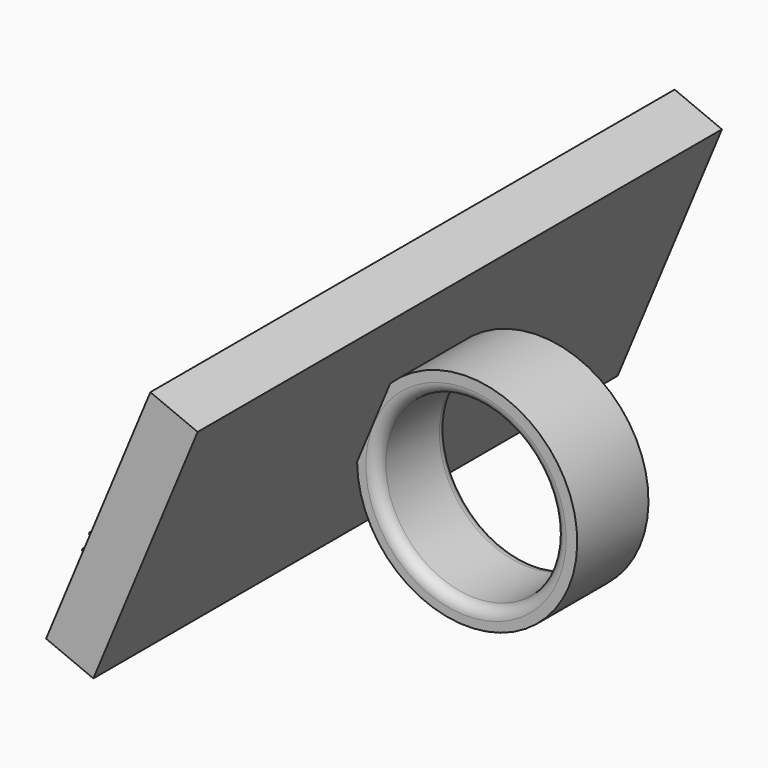
from build123d import *

# Parameters (mm, degrees)
F0_R           = 10.16
F1_DEPTH       = 10.16
F2_R           = 1.27
F3_R           = 1.27
F5_W           = 74.7877769172
F5_H           = 31.0049764812
F6_DEPTH       = 5.842
F7_TEXT_SIZE   = 4.4080810363
F7_TEXT_SIZE_2 = 4.4057197455
F7_TEXT_SIZE_3 = 4.3735069792
F7_TEXT_SIZE_4 = 4.335331121
F7_TEXT_SIZE_5 = 4.2736875912
F7_TEXT_SIZE_6 = 4.2982167037
F7_TEXT_SIZE_7 = 4.3517716727
F7_TEXT_SIZE_8 = 4.3960835481
F8_DEPTH       = 1.524


# Not quite as in the source:
# - Text() gives the source's letters only with a copy of the font that has no kerning and outlines rounded to 1/6400 em; it was checked with that copy


with BuildPart() as f1:
    # F0 (on Front) → F1 (new body)
    with BuildSketch(Plane.XZ):
        with BuildLine():
            Line((-8.6544063684, 9.0933511978), (-12.4330554948, 0))
            ThreePointArc((-12.4330554948, 0), (11.730902079, -4.7093204288), (-8.6544063684, 9.0933511978))
        make_face()
        Circle(F0_R, mode=Mode.SUBTRACT)
    extrude(amount=F1_DEPTH)

    # F2
    f2_edges = [f1.edges().sort_by_distance(p)[0] for p in [
        (-10.16, 0, 0),
    ]]
    fillet(f2_edges, radius=F2_R)

    # F3
    f3_edges = [f1.edges().sort_by_distance(p)[0] for p in [
        (-10.16, -10.16, 0),
    ]]
    fillet(f3_edges, radius=F3_R)

    # F5 (on offset) → F6 (join)
    with BuildSketch(Plane(origin=(-10.6023181655, 0, 4.4056849232), x_dir=(0, -1, 0), z_dir=(-0.9234459488, 0, 0.3837285234))):
        with Locations((5.2367541939, 0)):
            Rectangle(F5_W, F5_H)
    extrude(amount=F6_DEPTH)

    # F7 (on face) → F8 (join)
    with BuildSketch(Plane(origin=(-15.9970893984, 0, 6.6474269568), x_dir=(0, -1, 0), z_dir=(-0.9234459488, 0, 0.3837285234))):
        with Locations((-22.3117806017, 8.8225803338)):
            Text('Silhouette Ballroom Studios', F7_TEXT_SIZE, font='Open Sans', text_align=(TextAlign.LEFT, TextAlign.BOTTOM))
        with Locations((-27.9232524335, 2.3819217458)):
            Text('Tango', F7_TEXT_SIZE_2, font='Open Sans', text_align=(TextAlign.LEFT, TextAlign.BOTTOM))
        with Locations((-17.7410431206, -2.6636847761)):
            Text('Rumba', F7_TEXT_SIZE_3, font='Open Sans', text_align=(TextAlign.LEFT, TextAlign.BOTTOM))
        with Locations((1.3777401764, 2.4045574246)):
            Text('West Coast Swing', F7_TEXT_SIZE_4, font='Open Sans', text_align=(TextAlign.LEFT, TextAlign.BOTTOM))
        with Locations((-23.7387232482, -9.3680929567)):
            Text('Viennese Waltz', F7_TEXT_SIZE_5, font='Open Sans', text_align=(TextAlign.LEFT, TextAlign.BOTTOM))
        with Locations((9.2386431643, -4.645234294)):
            Text('Polka', F7_TEXT_SIZE_6, font='Open Sans', text_align=(TextAlign.LEFT, TextAlign.BOTTOM))
        with Locations((25.2182949334, -7.2010576259)):
            Text('Foxtrot', F7_TEXT_SIZE_7, font='Open Sans', text_align=(TextAlign.LEFT, TextAlign.BOTTOM))
        with Locations((17.3978812527, -13.1856857624)):
            Text('Samba', F7_TEXT_SIZE_8, font='Open Sans', text_align=(TextAlign.LEFT, TextAlign.BOTTOM))
    extrude(amount=F8_DEPTH)


solid = f1.part
